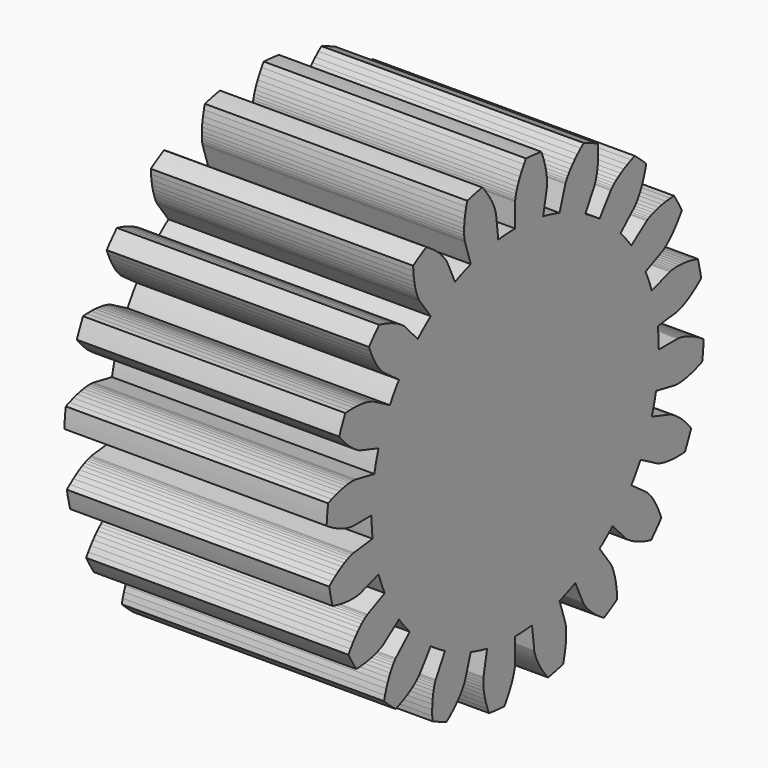
from build123d import *

# Parameters (mm, degrees)
F2_DEPTH = 12.7


# Not quite as in the source:
# - a variable given as a bare number and used for a length is read in inches; the dataset says mm whatever the document's units were


with BuildPart() as f2:
    # F1 (on Right) → F2 (new body)
    with BuildSketch(Plane.YZ):
        with BuildLine():
            ThreePointArc((8.5236223657, -1.6954539034), (8.6487623375, -0.8518287399), (8.69061, 0))
            ThreePointArc((8.69061, 0), (8.6755370945, 0.5116231949), (8.6303706627, 1.0214716817))
            ThreePointArc((8.6303706627, 1.0214716817), (8.4886913359, 1.8624772687), (8.2652612711, 2.6855461815))
            ThreePointArc((8.2652612711, 2.6855461815), (8.0928258242, 3.167470971), (7.8923181479, 3.6384085016))
            ThreePointArc((7.8923181479, 3.6384085016), (7.4976880821, 4.3944710257), (7.0308511815, 5.1082123914))
            ThreePointArc((7.0308511815, 5.1082123914), (6.7179323761, 5.5132646193), (6.3817105437, 5.8991925471))
            ThreePointArc((6.3817105437, 5.8991925471), (5.7727588794, 6.4963033405), (5.1082123914, 7.0308511815))
            ThreePointArc((5.1082123914, 7.0308511815), (4.6854409005, 7.3193815135), (4.2464166476, 7.582522524))
            ThreePointArc((4.2464166476, 7.582522524), (3.4827518165, 7.962232222), (2.6855461815, 8.2652612711))
            ThreePointArc((2.6855461815, 8.2652612711), (2.1943058241, 8.4090263481), (1.6954539034, 8.5236223657))
            ThreePointArc((1.6954539034, 8.5236223657), (0.8518287399, 8.6487623375), (0, 8.69061))
            ThreePointArc((0, 8.69061), (-0.5116231949, 8.6755370945), (-1.0214716817, 8.6303706627))
            ThreePointArc((-1.0214716817, 8.6303706627), (-1.8624772687, 8.4886913359), (-2.6855461815, 8.2652612711))
            ThreePointArc((-2.6855461815, 8.2652612711), (-3.167470971, 8.0928258242), (-3.6384085016, 7.8923181479))
            ThreePointArc((-3.6384085016, 7.8923181479), (-4.3944710257, 7.4976880821), (-5.1082123914, 7.0308511815))
            ThreePointArc((-5.1082123914, 7.0308511815), (-5.5132646193, 6.7179323761), (-5.8991925471, 6.3817105437))
            ThreePointArc((-5.8991925471, 6.3817105437), (-6.4963033405, 5.7727588794), (-7.0308511815, 5.1082123914))
            ThreePointArc((-7.0308511815, 5.1082123914), (-7.3193815135, 4.6854409005), (-7.582522524, 4.2464166476))
            ThreePointArc((-7.582522524, 4.2464166476), (-7.962232222, 3.4827518165), (-8.2652612711, 2.6855461815))
            ThreePointArc((-8.2652612711, 2.6855461815), (-8.4090263481, 2.1943058241), (-8.5236223657, 1.6954539034))
            ThreePointArc((-8.5236223657, 1.6954539034), (-8.6487623375, 0.8518287399), (-8.69061, 0))
            ThreePointArc((-8.69061, 0), (-8.6755370945, -0.5116231949), (-8.6303706627, -1.0214716817))
            ThreePointArc((-8.6303706627, -1.0214716817), (-8.4886913359, -1.8624772687), (-8.2652612711, -2.6855461815))
            ThreePointArc((-8.2652612711, -2.6855461815), (-8.0928258242, -3.167470971), (-7.8923181479, -3.6384085016))
            ThreePointArc((-7.8923181479, -3.6384085016), (-7.4976880821, -4.3944710257), (-7.0308511815, -5.1082123914))
            ThreePointArc((-7.0308511815, -5.1082123914), (-6.7179323761, -5.5132646193), (-6.3817105437, -5.8991925471))
            ThreePointArc((-6.3817105437, -5.8991925471), (-5.7727588794, -6.4963033405), (-5.1082123914, -7.0308511815))
            ThreePointArc((-5.1082123914, -7.0308511815), (-4.6854409005, -7.3193815135), (-4.2464166476, -7.582522524))
            ThreePointArc((-4.2464166476, -7.582522524), (-3.4827518165, -7.962232222), (-2.6855461815, -8.2652612711))
            ThreePointArc((-2.6855461815, -8.2652612711), (-2.1943058241, -8.4090263481), (-1.6954539034, -8.5236223657))
            ThreePointArc((-1.6954539034, -8.5236223657), (-0.8518287399, -8.6487623375), (0, -8.69061))
            ThreePointArc((0, -8.69061), (0.5116231949, -8.6755370945), (1.0214716817, -8.6303706627))
            ThreePointArc((1.0214716817, -8.6303706627), (1.8624772687, -8.4886913359), (2.6855461815, -8.2652612711))
            ThreePointArc((2.6855461815, -8.2652612711), (3.167470971, -8.0928258242), (3.6384085016, -7.8923181479))
            ThreePointArc((3.6384085016, -7.8923181479), (4.3944710257, -7.4976880821), (5.1082123914, -7.0308511815))
            ThreePointArc((5.1082123914, -7.0308511815), (5.5132646193, -6.7179323761), (5.8991925471, -6.3817105437))
            ThreePointArc((5.8991925471, -6.3817105437), (6.4963033405, -5.7727588794), (7.0308511815, -5.1082123914))
            ThreePointArc((7.0308511815, -5.1082123914), (7.3193815135, -4.6854409005), (7.582522524, -4.2464166476))
            ThreePointArc((7.582522524, -4.2464166476), (7.962232222, -3.4827518165), (8.2652612711, -2.6855461815))
            ThreePointArc((8.2652612711, -2.6855461815), (8.4090263481, -2.1943058241), (8.5236223657, -1.6954539034))
        make_face()
        with BuildLine():
            Line((-9.3549533207, -3.0396085912), (-8.2652612711, -2.6855461815))
            ThreePointArc((-8.2652612711, -2.6855461815), (-8.4886913359, -1.8624772687), (-8.6303706627, -1.0214716817))
            Line((-8.6303706627, -1.0214716817), (-9.7681987347, -1.1561425087))
            Line((-9.7681987347, -1.1561425087), (-9.780353193, -1.157993683))
            Line((-9.780353193, -1.157993683), (-9.8165326998, -1.1651615743))
            Line((-9.8165326998, -1.1651615743), (-9.8761758653, -1.180040537))
            Line((-9.8761758653, -1.180040537), (-9.9585426782, -1.2049790988))
            Line((-9.9585426782, -1.2049790988), (-10.0627178322, -1.2422681281))
            Line((-10.0627178322, -1.2422681281), (-10.1876147871, -1.2941292255))
            Line((-10.1876147871, -1.2941292255), (-10.3319805495, -1.3627033855))
            Line((-10.3319805495, -1.3627033855), (-10.4944011563, -1.4500399701))
            Line((-10.4944011563, -1.4500399701), (-10.6733078407, -1.5580860349))
            Line((-10.6733078407, -1.5580860349), (-10.8669838603, -1.6886760511))
            Line((-10.8669838603, -1.6886760511), (-11.0735719609, -1.8435220595))
            Line((-11.0735719609, -1.8435220595), (-11.2547256997, -1.994003366))
            ThreePointArc((-11.2547256997, -1.994003366), (-11.1644340235, -2.4495536195), (-11.0557112434, -2.901059962))
            Line((-11.0557112434, -2.901059962), (-10.8281972477, -2.9618767566))
            Line((-10.8281972477, -2.9618767566), (-10.5757578852, -3.0160089821))
            Line((-10.5757578852, -3.0160089821), (-10.3451995481, -3.0535190624))
            Line((-10.3451995481, -3.0535190624), (-10.1374921268, -3.0767393331))
            Line((-10.1374921268, -3.0767393331), (-9.9534266499, -3.0880544876))
            Line((-9.9534266499, -3.0880544876), (-9.7936126283, -3.0898895107))
            Line((-9.7936126283, -3.0898895107), (-9.6584761579, -3.0846974859))
            Line((-9.6584761579, -3.0846974859), (-9.5482587877, -3.0749473207))
            Line((-9.5482587877, -3.0749473207), (-9.4630171571, -3.0631114372))
            Line((-9.4630171571, -3.0631114372), (-9.4026234009, -3.0516534735))
            Line((-9.4026234009, -3.0516534735), (-9.3667663213, -3.0430160422))
            Line((-9.3667663213, -3.0430160422), (-9.3549533207, -3.0396085912))
        make_face()
        with BuildLine():
            Line((-7.9577986044, -5.7816791154), (-7.0308511815, -5.1082123914))
            ThreePointArc((-7.0308511815, -5.1082123914), (-7.4976880821, -4.3944710257), (-7.8923181479, -3.6384085016))
            Line((-7.8923181479, -3.6384085016), (-8.932841376, -4.1180962801))
            Line((-8.932841376, -4.1180962801), (-8.9438289085, -4.1236127857))
            Line((-8.9438289085, -4.1236127857), (-8.9760226639, -4.1416099379))
            Line((-8.9760226639, -4.1416099379), (-9.0281488328, -4.174191424))
            Line((-9.0281488328, -4.174191424), (-9.0987778875, -4.2233621507))
            Line((-9.0987778875, -4.2233621507), (-9.1863314028, -4.291018018))
            Line((-9.1863314028, -4.291018018), (-9.2890895052, -4.3789361342))
            Line((-9.2890895052, -4.3789361342), (-9.4051989235, -4.4887655099))
            Line((-9.4051989235, -4.4887655099), (-9.532681611, -4.6220182655))
            Line((-9.532681611, -4.6220182655), (-9.6694439088, -4.7800613854))
            Line((-9.6694439088, -4.7800613854), (-9.813286215, -4.9641090528))
            Line((-9.813286215, -4.9641090528), (-9.9619131262, -5.175215592))
            Line((-9.9619131262, -5.175215592), (-10.0876992889, -5.374311403))
            ThreePointArc((-10.0876992889, -5.374311403), (-9.8610540317, -5.7796637777), (-9.6181293903, -6.1754746402))
            Line((-9.6181293903, -6.1754746402), (-9.3829572991, -6.1630091578))
            Line((-9.3829572991, -6.1630091578), (-9.1261454208, -6.1364839106))
            Line((-9.1261454208, -6.1364839106), (-8.8952801597, -6.1009116725))
            Line((-8.8952801597, -6.1009116725), (-8.6905632048, -6.0588103392))
            Line((-8.6905632048, -6.0588103392), (-8.5120099586, -6.0126923302))
            Line((-8.5120099586, -6.0126923302), (-8.3594507387, -5.9650522923))
            Line((-8.3594507387, -5.9650522923), (-8.2325327418, -5.9183549173))
            Line((-8.2325327418, -5.9183549173), (-8.1307227604, -5.8750229187))
            Line((-8.1307227604, -5.8750229187), (-8.0533106413, -5.837425212))
            Line((-8.0533106413, -5.837425212), (-7.9994134714, -5.807865344))
            Line((-7.9994134714, -5.807865344), (-7.9679804752, -5.7885702118))
            Line((-7.9679804752, -5.7885702118), (-7.9577986044, -5.7816791154))
        make_face()
        with BuildLine():
            Line((-5.7816791154, -7.9577986044), (-5.1082123914, -7.0308511815))
            ThreePointArc((-5.1082123914, -7.0308511815), (-5.7727588794, -6.4963033405), (-6.3817105437, -5.8991925471))
            Line((-6.3817105437, -5.8991925471), (-7.2230752646, -6.6769420952))
            Line((-7.2230752646, -6.6769420952), (-7.231820335, -6.685583938))
            Line((-7.231820335, -6.685583938), (-7.2568769901, -6.7126486644))
            Line((-7.2568769901, -6.7126486644), (-7.2963836897, -6.7597433711))
            Line((-7.2963836897, -6.7597433711), (-7.3483613222, -6.8283330894))
            Line((-7.3483613222, -6.8283330894), (-7.4107228507, -6.9197331669))
            Line((-7.4107228507, -6.9197331669), (-7.4812834216, -7.0351022642))
            Line((-7.4812834216, -7.0351022642), (-7.5577708969, -7.1754359912))
            Line((-7.5577708969, -7.1754359912), (-7.6378367716, -7.3415612096))
            Line((-7.6378367716, -7.3415612096), (-7.7190674362, -7.5341310229))
            Line((-7.7190674362, -7.5341310229), (-7.7989957418, -7.7536204733))
            Line((-7.7989957418, -7.7536204733), (-7.8751128259, -8.0003229645))
            Line((-7.8751128259, -8.0003229645), (-7.9332185865, -8.2285443949))
            ThreePointArc((-7.9332185865, -8.2285443949), (-7.5924053653, -8.544020176), (-7.2390580191, -8.8453908334))
            Line((-7.2390580191, -8.8453908334), (-7.0192481152, -8.7608632825))
            Line((-7.0192481152, -8.7608632825), (-6.783202257, -8.6562770384))
            Line((-6.783202257, -8.6562770384), (-6.5746287721, -8.5511045405))
            Line((-6.5746287721, -8.5511045405), (-6.3929414057, -8.4478027751))
            Line((-6.3929414057, -8.4478027751), (-6.2373784259, -8.3487659546))
            Line((-6.2373784259, -8.3487659546), (-6.107007567, -8.2563141945))
            Line((-6.107007567, -8.2563141945), (-6.0007316615, -8.1726825338))
            Line((-6.0007316615, -8.1726825338), (-5.9172949393, -8.1000103397))
            Line((-5.9172949393, -8.1000103397), (-5.8552899692, -8.0403311354))
            Line((-5.8552899692, -8.0403311354), (-5.8131652162, -7.9955628889))
            Line((-5.8131652162, -7.9955628889), (-5.7892331841, -7.9674987976))
            Line((-5.7892331841, -7.9674987976), (-5.7816791154, -7.9577986044))
        make_face()
        with BuildLine():
            Line((-3.0396085912, -9.3549533207), (-2.6855461815, -8.2652612711))
            ThreePointArc((-2.6855461815, -8.2652612711), (-3.4827518165, -7.962232222), (-4.2464166476, -7.582522524))
            Line((-4.2464166476, -7.582522524), (-4.8062642203, -8.5822022969))
            Line((-4.8062642203, -8.5822022969), (-4.8119108001, -8.5931235533))
            Line((-4.8119108001, -8.5931235533), (-4.8273776348, -8.6266065699))
            Line((-4.8273776348, -8.6266065699), (-4.8503976742, -8.6836045392))
            Line((-4.8503976742, -8.6836045392), (-4.8786359517, -8.7648992095))
            Line((-4.8786359517, -8.7648992095), (-4.9097011125, -8.8710966209))
            Line((-4.9097011125, -8.8710966209), (-4.9411571916, -9.0026235682))
            Line((-4.9411571916, -9.0026235682), (-4.9705355968, -9.1597248034))
            Line((-4.9705355968, -9.1597248034), (-4.995347253, -9.3424609909))
            Line((-4.995347253, -9.3424609909), (-5.013094861, -9.5507074225))
            Line((-5.013094861, -9.5507074225), (-5.0212852266, -9.7841534993))
            Line((-5.0212852266, -9.7841534993), (-5.0174416132, -10.0423029836))
            Line((-5.0174416132, -10.0423029836), (-5.0021791749, -10.2773101297))
            ThreePointArc((-5.0021791749, -10.2773101297), (-4.5805591624, -10.4720283498), (-4.1513772115, -10.6494585425))
            Line((-4.1513772115, -10.6494585425), (-3.9684460198, -10.5011430685))
            Line((-3.9684460198, -10.5011430685), (-3.776271995, -10.328733458))
            Line((-3.776271995, -10.328733458), (-3.6104069123, -10.1642557171))
            Line((-3.6104069123, -10.1642557171), (-3.4695339596, -10.009865416))
            Line((-3.4695339596, -10.009865416), (-3.3521888346, -9.8676041981))
            Line((-3.3521888346, -9.8676041981), (-3.2567679447, -9.7393905383))
            Line((-3.2567679447, -9.7393905383), (-3.1815371566, -9.6270110415))
            Line((-3.1815371566, -9.6270110415), (-3.1246410612, -9.5321123126))
            Line((-3.1246410612, -9.5321123126), (-3.0841127188, -9.456193427))
            Line((-3.0841127188, -9.456193427), (-3.0578838469, -9.4005990298))
            Line((-3.0578838469, -9.4005990298), (-3.043795413, -9.3665130884))
            Line((-3.043795413, -9.3665130884), (-3.0396085912, -9.3549533207))
        make_face()
        with BuildLine():
            Line((0, -9.8363800262), (0, -8.69061))
            ThreePointArc((0, -8.69061), (-0.8518287399, -8.6487623375), (-1.6954539034, -8.5236223657))
            Line((-1.6954539034, -8.5236223657), (-1.9189825468, -9.6473767422))
            Line((-1.9189825468, -9.6473767422), (-1.9209779096, -9.6595083634))
            Line((-1.9209779096, -9.6595083634), (-1.9253409223, -9.6961321192))
            Line((-1.9253409223, -9.6961321192), (-1.9296209396, -9.7574539927))
            Line((-1.9296209396, -9.7574539927), (-1.9313557028, -9.8434959263))
            Line((-1.9313557028, -9.8434959263), (-1.9280836215, -9.9540953291))
            Line((-1.9280836215, -9.9540953291), (-1.9173560686, -10.0889053524))
            Line((-1.9173560686, -10.0889053524), (-1.8967496408, -10.2473959323))
            Line((-1.8967496408, -10.2473959323), (-1.8638783407, -10.4288555976))
            Line((-1.8638783407, -10.4288555976), (-1.8164056325, -10.6323940358))
            Line((-1.8164056325, -10.6323940358), (-1.7520563281, -10.8569454106))
            Line((-1.7520563281, -10.8569454106), (-1.6686282567, -11.101272418))
            Line((-1.6686282567, -11.101272418), (-1.5814916135, -11.3200611428))
            ThreePointArc((-1.5814916135, -11.3200611428), (-1.120335914, -11.3749614259), (-0.657330678, -11.4110830503))
            Line((-0.657330678, -11.4110830503), (-0.5291847781, -11.2134978052))
            Line((-0.5291847781, -11.2134978052), (-0.3996939192, -10.9901414821))
            Line((-0.3996939192, -10.9901414821), (-0.2927732686, -10.7824587255))
            Line((-0.2927732686, -10.7824587255), (-0.2065043558, -10.5920926872))
            Line((-0.2065043558, -10.5920926872), (-0.138863644, -10.4205325911))
            Line((-0.138863644, -10.4205325911), (-0.0877331847, -10.2691074778))
            Line((-0.0877331847, -10.2691074778), (-0.0509116278, -10.1389806331))
            Line((-0.0509116278, -10.1389806331), (-0.0261255455, -10.0311447182))
            Line((-0.0261255455, -10.0311447182), (-0.0110410272, -9.9464176208))
            Line((-0.0110410272, -9.9464176208), (-0.0032755011, -9.8854390399))
            Line((-0.0032755011, -9.8854390399), (-0.0004097394, -9.8486678177))
            Line((-0.0004097394, -9.8486678177), (0, -9.8363800262))
        make_face()
        with BuildLine():
            Line((3.0396085912, -9.3549533207), (2.6855461815, -8.2652612711))
            ThreePointArc((2.6855461815, -8.2652612711), (1.8624772687, -8.4886913359), (1.0214716817, -8.6303706627))
            Line((1.0214716817, -8.6303706627), (1.1561425087, -9.7681987347))
            Line((1.1561425087, -9.7681987347), (1.157993683, -9.780353193))
            Line((1.157993683, -9.780353193), (1.1651615743, -9.8165326998))
            Line((1.1651615743, -9.8165326998), (1.180040537, -9.8761758653))
            Line((1.180040537, -9.8761758653), (1.2049790988, -9.9585426782))
            Line((1.2049790988, -9.9585426782), (1.2422681281, -10.0627178322))
            Line((1.2422681281, -10.0627178322), (1.2941292255, -10.1876147871))
            Line((1.2941292255, -10.1876147871), (1.3627033855, -10.3319805495))
            Line((1.3627033855, -10.3319805495), (1.4500399701, -10.4944011563))
            Line((1.4500399701, -10.4944011563), (1.5580860349, -10.6733078407))
            Line((1.5580860349, -10.6733078407), (1.6886760511, -10.8669838603))
            Line((1.6886760511, -10.8669838603), (1.8435220595, -11.0735719609))
            Line((1.8435220595, -11.0735719609), (1.994003366, -11.2547256997))
            ThreePointArc((1.994003366, -11.2547256997), (2.4495536195, -11.1644340235), (2.901059962, -11.0557112434))
            Line((2.901059962, -11.0557112434), (2.9618767566, -10.8281972477))
            Line((2.9618767566, -10.8281972477), (3.0160089821, -10.5757578852))
            Line((3.0160089821, -10.5757578852), (3.0535190624, -10.3451995481))
            Line((3.0535190624, -10.3451995481), (3.0767393331, -10.1374921268))
            Line((3.0767393331, -10.1374921268), (3.0880544876, -9.9534266499))
            Line((3.0880544876, -9.9534266499), (3.0898895107, -9.7936126283))
            Line((3.0898895107, -9.7936126283), (3.0846974859, -9.6584761579))
            Line((3.0846974859, -9.6584761579), (3.0749473207, -9.5482587877))
            Line((3.0749473207, -9.5482587877), (3.0631114372, -9.4630171571))
            Line((3.0631114372, -9.4630171571), (3.0516534735, -9.4026234009))
            Line((3.0516534735, -9.4026234009), (3.0430160422, -9.3667663213))
            Line((3.0430160422, -9.3667663213), (3.0396085912, -9.3549533207))
        make_face()
        with BuildLine():
            Line((5.7816791154, -7.9577986044), (5.1082123914, -7.0308511815))
            ThreePointArc((5.1082123914, -7.0308511815), (4.3944710257, -7.4976880821), (3.6384085016, -7.8923181479))
            Line((3.6384085016, -7.8923181479), (4.1180962801, -8.932841376))
            Line((4.1180962801, -8.932841376), (4.1236127857, -8.9438289085))
            Line((4.1236127857, -8.9438289085), (4.1416099379, -8.9760226639))
            Line((4.1416099379, -8.9760226639), (4.174191424, -9.0281488328))
            Line((4.174191424, -9.0281488328), (4.2233621507, -9.0987778875))
            Line((4.2233621507, -9.0987778875), (4.291018018, -9.1863314028))
            Line((4.291018018, -9.1863314028), (4.3789361342, -9.2890895052))
            Line((4.3789361342, -9.2890895052), (4.4887655099, -9.4051989235))
            Line((4.4887655099, -9.4051989235), (4.6220182655, -9.532681611))
            Line((4.6220182655, -9.532681611), (4.7800613854, -9.6694439088))
            Line((4.7800613854, -9.6694439088), (4.9641090528, -9.813286215))
            Line((4.9641090528, -9.813286215), (5.175215592, -9.9619131262))
            Line((5.175215592, -9.9619131262), (5.374311403, -10.0876992889))
            ThreePointArc((5.374311403, -10.0876992889), (5.7796637777, -9.8610540317), (6.1754746402, -9.6181293903))
            Line((6.1754746402, -9.6181293903), (6.1630091578, -9.3829572991))
            Line((6.1630091578, -9.3829572991), (6.1364839106, -9.1261454208))
            Line((6.1364839106, -9.1261454208), (6.1009116725, -8.8952801597))
            Line((6.1009116725, -8.8952801597), (6.0588103392, -8.6905632048))
            Line((6.0588103392, -8.6905632048), (6.0126923302, -8.5120099586))
            Line((6.0126923302, -8.5120099586), (5.9650522923, -8.3594507387))
            Line((5.9650522923, -8.3594507387), (5.9183549173, -8.2325327418))
            Line((5.9183549173, -8.2325327418), (5.8750229187, -8.1307227604))
            Line((5.8750229187, -8.1307227604), (5.837425212, -8.0533106413))
            Line((5.837425212, -8.0533106413), (5.807865344, -7.9994134714))
            Line((5.807865344, -7.9994134714), (5.7885702118, -7.9679804752))
            Line((5.7885702118, -7.9679804752), (5.7816791154, -7.9577986044))
        make_face()
        with BuildLine():
            Line((7.9577986044, -5.7816791154), (7.0308511815, -5.1082123914))
            ThreePointArc((7.0308511815, -5.1082123914), (6.4963033405, -5.7727588794), (5.8991925471, -6.3817105437))
            Line((5.8991925471, -6.3817105437), (6.6769420952, -7.2230752646))
            Line((6.6769420952, -7.2230752646), (6.685583938, -7.231820335))
            Line((6.685583938, -7.231820335), (6.7126486644, -7.2568769901))
            Line((6.7126486644, -7.2568769901), (6.7597433711, -7.2963836897))
            Line((6.7597433711, -7.2963836897), (6.8283330894, -7.3483613222))
            Line((6.8283330894, -7.3483613222), (6.9197331669, -7.4107228507))
            Line((6.9197331669, -7.4107228507), (7.0351022642, -7.4812834216))
            Line((7.0351022642, -7.4812834216), (7.1754359912, -7.5577708969))
            Line((7.1754359912, -7.5577708969), (7.3415612096, -7.6378367716))
            Line((7.3415612096, -7.6378367716), (7.5341310229, -7.7190674362))
            Line((7.5341310229, -7.7190674362), (7.7536204733, -7.7989957418))
            Line((7.7536204733, -7.7989957418), (8.0003229645, -7.8751128259))
            Line((8.0003229645, -7.8751128259), (8.2285443949, -7.9332185865))
            ThreePointArc((8.2285443949, -7.9332185865), (8.544020176, -7.5924053653), (8.8453908334, -7.2390580191))
            Line((8.8453908334, -7.2390580191), (8.7608632825, -7.0192481152))
            Line((8.7608632825, -7.0192481152), (8.6562770384, -6.783202257))
            Line((8.6562770384, -6.783202257), (8.5511045405, -6.5746287721))
            Line((8.5511045405, -6.5746287721), (8.4478027751, -6.3929414057))
            Line((8.4478027751, -6.3929414057), (8.3487659546, -6.2373784259))
            Line((8.3487659546, -6.2373784259), (8.2563141945, -6.107007567))
            Line((8.2563141945, -6.107007567), (8.1726825338, -6.0007316615))
            Line((8.1726825338, -6.0007316615), (8.1000103397, -5.9172949393))
            Line((8.1000103397, -5.9172949393), (8.0403311354, -5.8552899692))
            Line((8.0403311354, -5.8552899692), (7.9955628889, -5.8131652162))
            Line((7.9955628889, -5.8131652162), (7.9674987976, -5.7892331841))
            Line((7.9674987976, -5.7892331841), (7.9577986044, -5.7816791154))
        make_face()
        with BuildLine():
            Line((9.3549533207, -3.0396085912), (8.2652612711, -2.6855461815))
            ThreePointArc((8.2652612711, -2.6855461815), (7.962232222, -3.4827518165), (7.582522524, -4.2464166476))
            Line((7.582522524, -4.2464166476), (8.5822022969, -4.8062642203))
            Line((8.5822022969, -4.8062642203), (8.5931235533, -4.8119108001))
            Line((8.5931235533, -4.8119108001), (8.6266065699, -4.8273776348))
            Line((8.6266065699, -4.8273776348), (8.6836045392, -4.8503976742))
            Line((8.6836045392, -4.8503976742), (8.7648992095, -4.8786359517))
            Line((8.7648992095, -4.8786359517), (8.8710966209, -4.9097011125))
            Line((8.8710966209, -4.9097011125), (9.0026235682, -4.9411571916))
            Line((9.0026235682, -4.9411571916), (9.1597248034, -4.9705355968))
            Line((9.1597248034, -4.9705355968), (9.3424609909, -4.995347253))
            Line((9.3424609909, -4.995347253), (9.5507074225, -5.013094861))
            Line((9.5507074225, -5.013094861), (9.7841534993, -5.0212852266))
            Line((9.7841534993, -5.0212852266), (10.0423029836, -5.0174416132))
            Line((10.0423029836, -5.0174416132), (10.2773101297, -5.0021791749))
            ThreePointArc((10.2773101297, -5.0021791749), (10.4720283498, -4.5805591624), (10.6494585425, -4.1513772115))
            Line((10.6494585425, -4.1513772115), (10.5011430685, -3.9684460198))
            Line((10.5011430685, -3.9684460198), (10.328733458, -3.776271995))
            Line((10.328733458, -3.776271995), (10.1642557171, -3.6104069123))
            Line((10.1642557171, -3.6104069123), (10.009865416, -3.4695339596))
            Line((10.009865416, -3.4695339596), (9.8676041981, -3.3521888346))
            Line((9.8676041981, -3.3521888346), (9.7393905383, -3.2567679447))
            Line((9.7393905383, -3.2567679447), (9.6270110415, -3.1815371566))
            Line((9.6270110415, -3.1815371566), (9.5321123126, -3.1246410612))
            Line((9.5321123126, -3.1246410612), (9.456193427, -3.0841127188))
            Line((9.456193427, -3.0841127188), (9.4005990298, -3.0578838469))
            Line((9.4005990298, -3.0578838469), (9.3665130884, -3.043795413))
            Line((9.3665130884, -3.043795413), (9.3549533207, -3.0396085912))
        make_face()
        with BuildLine():
            Line((9.8363800262, 0), (8.69061, 0))
            ThreePointArc((8.69061, 0), (8.6487623375, -0.8518287399), (8.5236223657, -1.6954539034))
            Line((8.5236223657, -1.6954539034), (9.6473767422, -1.9189825468))
            Line((9.6473767422, -1.9189825468), (9.6595083634, -1.9209779096))
            Line((9.6595083634, -1.9209779096), (9.6961321192, -1.9253409223))
            Line((9.6961321192, -1.9253409223), (9.7574539927, -1.9296209396))
            Line((9.7574539927, -1.9296209396), (9.8434959263, -1.9313557028))
            Line((9.8434959263, -1.9313557028), (9.9540953291, -1.9280836215))
            Line((9.9540953291, -1.9280836215), (10.0889053524, -1.9173560686))
            Line((10.0889053524, -1.9173560686), (10.2473959323, -1.8967496408))
            Line((10.2473959323, -1.8967496408), (10.4288555976, -1.8638783407))
            Line((10.4288555976, -1.8638783407), (10.6323940358, -1.8164056325))
            Line((10.6323940358, -1.8164056325), (10.8569454106, -1.7520563281))
            Line((10.8569454106, -1.7520563281), (11.101272418, -1.6686282567))
            Line((11.101272418, -1.6686282567), (11.3200611428, -1.5814916135))
            ThreePointArc((11.3200611428, -1.5814916135), (11.3749614259, -1.120335914), (11.4110830503, -0.657330678))
            Line((11.4110830503, -0.657330678), (11.2134978052, -0.5291847781))
            Line((11.2134978052, -0.5291847781), (10.9901414821, -0.3996939192))
            Line((10.9901414821, -0.3996939192), (10.7824587255, -0.2927732686))
            Line((10.7824587255, -0.2927732686), (10.5920926872, -0.2065043558))
            Line((10.5920926872, -0.2065043558), (10.4205325911, -0.138863644))
            Line((10.4205325911, -0.138863644), (10.2691074778, -0.0877331847))
            Line((10.2691074778, -0.0877331847), (10.1389806331, -0.0509116278))
            Line((10.1389806331, -0.0509116278), (10.0311447182, -0.0261255455))
            Line((10.0311447182, -0.0261255455), (9.9464176208, -0.0110410272))
            Line((9.9464176208, -0.0110410272), (9.8854390399, -0.0032755011))
            Line((9.8854390399, -0.0032755011), (9.8486678177, -0.0004097394))
            Line((9.8486678177, -0.0004097394), (9.8363800262, 0))
        make_face()
        with BuildLine():
            ThreePointArc((8.2652612711, 2.6855461815), (8.4886913359, 1.8624772687), (8.6303706627, 1.0214716817))
            Line((8.6303706627, 1.0214716817), (9.7681987347, 1.1561425087))
            Line((9.7681987347, 1.1561425087), (9.780353193, 1.157993683))
            Line((9.780353193, 1.157993683), (9.8165326998, 1.1651615743))
            Line((9.8165326998, 1.1651615743), (9.8761758653, 1.180040537))
            Line((9.8761758653, 1.180040537), (9.9585426782, 1.2049790988))
            Line((9.9585426782, 1.2049790988), (10.0627178322, 1.2422681281))
            Line((10.0627178322, 1.2422681281), (10.1876147871, 1.2941292255))
            Line((10.1876147871, 1.2941292255), (10.3319805495, 1.3627033855))
            Line((10.3319805495, 1.3627033855), (10.4944011563, 1.4500399701))
            Line((10.4944011563, 1.4500399701), (10.6733078407, 1.5580860349))
            Line((10.6733078407, 1.5580860349), (10.8669838603, 1.6886760511))
            Line((10.8669838603, 1.6886760511), (11.0735719609, 1.8435220595))
            Line((11.0735719609, 1.8435220595), (11.2547256997, 1.994003366))
            ThreePointArc((11.2547256997, 1.994003366), (11.1644340235, 2.4495536195), (11.0557112434, 2.901059962))
            Line((11.0557112434, 2.901059962), (10.8281972477, 2.9618767566))
            Line((10.8281972477, 2.9618767566), (10.5757578852, 3.0160089821))
            Line((10.5757578852, 3.0160089821), (10.3451995481, 3.0535190624))
            Line((10.3451995481, 3.0535190624), (10.1374921268, 3.0767393331))
            Line((10.1374921268, 3.0767393331), (9.9534266499, 3.0880544876))
            Line((9.9534266499, 3.0880544876), (9.7936126283, 3.0898895107))
            Line((9.7936126283, 3.0898895107), (9.6584761579, 3.0846974859))
            Line((9.6584761579, 3.0846974859), (9.5482587877, 3.0749473207))
            Line((9.5482587877, 3.0749473207), (9.4630171571, 3.0631114372))
            Line((9.4630171571, 3.0631114372), (9.4026234009, 3.0516534735))
            Line((9.4026234009, 3.0516534735), (9.3667663213, 3.0430160422))
            Line((9.3667663213, 3.0430160422), (9.3549533207, 3.0396085912))
            Line((9.3549533207, 3.0396085912), (8.2652612711, 2.6855461815))
        make_face()
        with BuildLine():
            ThreePointArc((7.0308511815, 5.1082123914), (7.4976880821, 4.3944710257), (7.8923181479, 3.6384085016))
            Line((7.8923181479, 3.6384085016), (8.932841376, 4.1180962801))
            Line((8.932841376, 4.1180962801), (8.9438289085, 4.1236127857))
            Line((8.9438289085, 4.1236127857), (8.9760226639, 4.1416099379))
            Line((8.9760226639, 4.1416099379), (9.0281488328, 4.174191424))
            Line((9.0281488328, 4.174191424), (9.0987778875, 4.2233621507))
            Line((9.0987778875, 4.2233621507), (9.1863314028, 4.291018018))
            Line((9.1863314028, 4.291018018), (9.2890895052, 4.3789361342))
            Line((9.2890895052, 4.3789361342), (9.4051989235, 4.4887655099))
            Line((9.4051989235, 4.4887655099), (9.532681611, 4.6220182655))
            Line((9.532681611, 4.6220182655), (9.6694439088, 4.7800613854))
            Line((9.6694439088, 4.7800613854), (9.813286215, 4.9641090528))
            Line((9.813286215, 4.9641090528), (9.9619131262, 5.175215592))
            Line((9.9619131262, 5.175215592), (10.0876992889, 5.374311403))
            ThreePointArc((10.0876992889, 5.374311403), (9.8610540317, 5.7796637777), (9.6181293903, 6.1754746402))
            Line((9.6181293903, 6.1754746402), (9.3829572991, 6.1630091578))
            Line((9.3829572991, 6.1630091578), (9.1261454208, 6.1364839106))
            Line((9.1261454208, 6.1364839106), (8.8952801597, 6.1009116725))
            Line((8.8952801597, 6.1009116725), (8.6905632048, 6.0588103392))
            Line((8.6905632048, 6.0588103392), (8.5120099586, 6.0126923302))
            Line((8.5120099586, 6.0126923302), (8.3594507387, 5.9650522923))
            Line((8.3594507387, 5.9650522923), (8.2325327418, 5.9183549173))
            Line((8.2325327418, 5.9183549173), (8.1307227604, 5.8750229187))
            Line((8.1307227604, 5.8750229187), (8.0533106413, 5.837425212))
            Line((8.0533106413, 5.837425212), (7.9994134714, 5.807865344))
            Line((7.9994134714, 5.807865344), (7.9679804752, 5.7885702118))
            Line((7.9679804752, 5.7885702118), (7.9577986044, 5.7816791154))
            Line((7.9577986044, 5.7816791154), (7.0308511815, 5.1082123914))
        make_face()
        with BuildLine():
            ThreePointArc((5.1082123914, 7.0308511815), (5.7727588794, 6.4963033405), (6.3817105437, 5.8991925471))
            Line((6.3817105437, 5.8991925471), (7.2230752646, 6.6769420952))
            Line((7.2230752646, 6.6769420952), (7.231820335, 6.685583938))
            Line((7.231820335, 6.685583938), (7.2568769901, 6.7126486644))
            Line((7.2568769901, 6.7126486644), (7.2963836897, 6.7597433711))
            Line((7.2963836897, 6.7597433711), (7.3483613222, 6.8283330894))
            Line((7.3483613222, 6.8283330894), (7.4107228507, 6.9197331669))
            Line((7.4107228507, 6.9197331669), (7.4812834216, 7.0351022642))
            Line((7.4812834216, 7.0351022642), (7.5577708969, 7.1754359912))
            Line((7.5577708969, 7.1754359912), (7.6378367716, 7.3415612096))
            Line((7.6378367716, 7.3415612096), (7.7190674362, 7.5341310229))
            Line((7.7190674362, 7.5341310229), (7.7989957418, 7.7536204733))
            Line((7.7989957418, 7.7536204733), (7.8751128259, 8.0003229645))
            Line((7.8751128259, 8.0003229645), (7.9332185865, 8.2285443949))
            ThreePointArc((7.9332185865, 8.2285443949), (7.5924053653, 8.544020176), (7.2390580191, 8.8453908334))
            Line((7.2390580191, 8.8453908334), (7.0192481152, 8.7608632825))
            Line((7.0192481152, 8.7608632825), (6.783202257, 8.6562770384))
            Line((6.783202257, 8.6562770384), (6.5746287721, 8.5511045405))
            Line((6.5746287721, 8.5511045405), (6.3929414057, 8.4478027751))
            Line((6.3929414057, 8.4478027751), (6.2373784259, 8.3487659546))
            Line((6.2373784259, 8.3487659546), (6.107007567, 8.2563141945))
            Line((6.107007567, 8.2563141945), (6.0007316615, 8.1726825338))
            Line((6.0007316615, 8.1726825338), (5.9172949393, 8.1000103397))
            Line((5.9172949393, 8.1000103397), (5.8552899692, 8.0403311354))
            Line((5.8552899692, 8.0403311354), (5.8131652162, 7.9955628889))
            Line((5.8131652162, 7.9955628889), (5.7892331841, 7.9674987976))
            Line((5.7892331841, 7.9674987976), (5.7816791154, 7.9577986044))
            Line((5.7816791154, 7.9577986044), (5.1082123914, 7.0308511815))
        make_face()
        with BuildLine():
            ThreePointArc((2.6855461815, 8.2652612711), (3.4827518165, 7.962232222), (4.2464166476, 7.582522524))
            Line((4.2464166476, 7.582522524), (4.8062642203, 8.5822022969))
            Line((4.8062642203, 8.5822022969), (4.8119108001, 8.5931235533))
            Line((4.8119108001, 8.5931235533), (4.8273776348, 8.6266065699))
            Line((4.8273776348, 8.6266065699), (4.8503976742, 8.6836045392))
            Line((4.8503976742, 8.6836045392), (4.8786359517, 8.7648992095))
            Line((4.8786359517, 8.7648992095), (4.9097011125, 8.8710966209))
            Line((4.9097011125, 8.8710966209), (4.9411571916, 9.0026235682))
            Line((4.9411571916, 9.0026235682), (4.9705355968, 9.1597248034))
            Line((4.9705355968, 9.1597248034), (4.995347253, 9.3424609909))
            Line((4.995347253, 9.3424609909), (5.013094861, 9.5507074225))
            Line((5.013094861, 9.5507074225), (5.0212852266, 9.7841534993))
            Line((5.0212852266, 9.7841534993), (5.0174416132, 10.0423029836))
            Line((5.0174416132, 10.0423029836), (5.0021791749, 10.2773101297))
            ThreePointArc((5.0021791749, 10.2773101297), (4.5805591624, 10.4720283498), (4.1513772115, 10.6494585425))
            Line((4.1513772115, 10.6494585425), (3.9684460198, 10.5011430685))
            Line((3.9684460198, 10.5011430685), (3.776271995, 10.328733458))
            Line((3.776271995, 10.328733458), (3.6104069123, 10.1642557171))
            Line((3.6104069123, 10.1642557171), (3.4695339596, 10.009865416))
            Line((3.4695339596, 10.009865416), (3.3521888346, 9.8676041981))
            Line((3.3521888346, 9.8676041981), (3.2567679447, 9.7393905383))
            Line((3.2567679447, 9.7393905383), (3.1815371566, 9.6270110415))
            Line((3.1815371566, 9.6270110415), (3.1246410612, 9.5321123126))
            Line((3.1246410612, 9.5321123126), (3.0841127188, 9.456193427))
            Line((3.0841127188, 9.456193427), (3.0578838469, 9.4005990298))
            Line((3.0578838469, 9.4005990298), (3.043795413, 9.3665130884))
            Line((3.043795413, 9.3665130884), (3.0396085912, 9.3549533207))
            Line((3.0396085912, 9.3549533207), (2.6855461815, 8.2652612711))
        make_face()
        with BuildLine():
            ThreePointArc((0, 8.69061), (0.8518287399, 8.6487623375), (1.6954539034, 8.5236223657))
            Line((1.6954539034, 8.5236223657), (1.9189825468, 9.6473767422))
            Line((1.9189825468, 9.6473767422), (1.9209779096, 9.6595083634))
            Line((1.9209779096, 9.6595083634), (1.9253409223, 9.6961321192))
            Line((1.9253409223, 9.6961321192), (1.9296209396, 9.7574539927))
            Line((1.9296209396, 9.7574539927), (1.9313557028, 9.8434959263))
            Line((1.9313557028, 9.8434959263), (1.9280836215, 9.9540953291))
            Line((1.9280836215, 9.9540953291), (1.9173560686, 10.0889053524))
            Line((1.9173560686, 10.0889053524), (1.8967496408, 10.2473959323))
            Line((1.8967496408, 10.2473959323), (1.8638783407, 10.4288555976))
            Line((1.8638783407, 10.4288555976), (1.8164056325, 10.6323940358))
            Line((1.8164056325, 10.6323940358), (1.7520563281, 10.8569454106))
            Line((1.7520563281, 10.8569454106), (1.6686282567, 11.101272418))
            Line((1.6686282567, 11.101272418), (1.5814916135, 11.3200611428))
            ThreePointArc((1.5814916135, 11.3200611428), (1.120335914, 11.3749614259), (0.657330678, 11.4110830503))
            Line((0.657330678, 11.4110830503), (0.5291847781, 11.2134978052))
            Line((0.5291847781, 11.2134978052), (0.3996939192, 10.9901414821))
            Line((0.3996939192, 10.9901414821), (0.2927732686, 10.7824587255))
            Line((0.2927732686, 10.7824587255), (0.2065043558, 10.5920926872))
            Line((0.2065043558, 10.5920926872), (0.138863644, 10.4205325911))
            Line((0.138863644, 10.4205325911), (0.0877331847, 10.2691074778))
            Line((0.0877331847, 10.2691074778), (0.0509116278, 10.1389806331))
            Line((0.0509116278, 10.1389806331), (0.0261255455, 10.0311447182))
            Line((0.0261255455, 10.0311447182), (0.0110410272, 9.9464176208))
            Line((0.0110410272, 9.9464176208), (0.0032755011, 9.8854390399))
            Line((0.0032755011, 9.8854390399), (0.0004097394, 9.8486678177))
            Line((0.0004097394, 9.8486678177), (0, 9.8363800262))
            Line((0, 9.8363800262), (0, 8.69061))
        make_face()
        with BuildLine():
            ThreePointArc((-2.6855461815, 8.2652612711), (-1.8624772687, 8.4886913359), (-1.0214716817, 8.6303706627))
            Line((-1.0214716817, 8.6303706627), (-1.1561425087, 9.7681987347))
            Line((-1.1561425087, 9.7681987347), (-1.157993683, 9.780353193))
            Line((-1.157993683, 9.780353193), (-1.1651615743, 9.8165326998))
            Line((-1.1651615743, 9.8165326998), (-1.180040537, 9.8761758653))
            Line((-1.180040537, 9.8761758653), (-1.2049790988, 9.9585426782))
            Line((-1.2049790988, 9.9585426782), (-1.2422681281, 10.0627178322))
            Line((-1.2422681281, 10.0627178322), (-1.2941292255, 10.1876147871))
            Line((-1.2941292255, 10.1876147871), (-1.3627033855, 10.3319805495))
            Line((-1.3627033855, 10.3319805495), (-1.4500399701, 10.4944011563))
            Line((-1.4500399701, 10.4944011563), (-1.5580860349, 10.6733078407))
            Line((-1.5580860349, 10.6733078407), (-1.6886760511, 10.8669838603))
            Line((-1.6886760511, 10.8669838603), (-1.8435220595, 11.0735719609))
            Line((-1.8435220595, 11.0735719609), (-1.994003366, 11.2547256997))
            ThreePointArc((-1.994003366, 11.2547256997), (-2.4495536195, 11.1644340235), (-2.901059962, 11.0557112434))
            Line((-2.901059962, 11.0557112434), (-2.9618767566, 10.8281972477))
            Line((-2.9618767566, 10.8281972477), (-3.0160089821, 10.5757578852))
            Line((-3.0160089821, 10.5757578852), (-3.0535190624, 10.3451995481))
            Line((-3.0535190624, 10.3451995481), (-3.0767393331, 10.1374921268))
            Line((-3.0767393331, 10.1374921268), (-3.0880544876, 9.9534266499))
            Line((-3.0880544876, 9.9534266499), (-3.0898895107, 9.7936126283))
            Line((-3.0898895107, 9.7936126283), (-3.0846974859, 9.6584761579))
            Line((-3.0846974859, 9.6584761579), (-3.0749473207, 9.5482587877))
            Line((-3.0749473207, 9.5482587877), (-3.0631114372, 9.4630171571))
            Line((-3.0631114372, 9.4630171571), (-3.0516534735, 9.4026234009))
            Line((-3.0516534735, 9.4026234009), (-3.0430160422, 9.3667663213))
            Line((-3.0430160422, 9.3667663213), (-3.0396085912, 9.3549533207))
            Line((-3.0396085912, 9.3549533207), (-2.6855461815, 8.2652612711))
        make_face()
        with BuildLine():
            ThreePointArc((-5.1082123914, 7.0308511815), (-4.3944710257, 7.4976880821), (-3.6384085016, 7.8923181479))
            Line((-3.6384085016, 7.8923181479), (-4.1180962801, 8.932841376))
            Line((-4.1180962801, 8.932841376), (-4.1236127857, 8.9438289085))
            Line((-4.1236127857, 8.9438289085), (-4.1416099379, 8.9760226639))
            Line((-4.1416099379, 8.9760226639), (-4.174191424, 9.0281488328))
            Line((-4.174191424, 9.0281488328), (-4.2233621507, 9.0987778875))
            Line((-4.2233621507, 9.0987778875), (-4.291018018, 9.1863314028))
            Line((-4.291018018, 9.1863314028), (-4.3789361342, 9.2890895052))
            Line((-4.3789361342, 9.2890895052), (-4.4887655099, 9.4051989235))
            Line((-4.4887655099, 9.4051989235), (-4.6220182655, 9.532681611))
            Line((-4.6220182655, 9.532681611), (-4.7800613854, 9.6694439088))
            Line((-4.7800613854, 9.6694439088), (-4.9641090528, 9.813286215))
            Line((-4.9641090528, 9.813286215), (-5.175215592, 9.9619131262))
            Line((-5.175215592, 9.9619131262), (-5.374311403, 10.0876992889))
            ThreePointArc((-5.374311403, 10.0876992889), (-5.7796637777, 9.8610540317), (-6.1754746402, 9.6181293903))
            Line((-6.1754746402, 9.6181293903), (-6.1630091578, 9.3829572991))
            Line((-6.1630091578, 9.3829572991), (-6.1364839106, 9.1261454208))
            Line((-6.1364839106, 9.1261454208), (-6.1009116725, 8.8952801597))
            Line((-6.1009116725, 8.8952801597), (-6.0588103392, 8.6905632048))
            Line((-6.0588103392, 8.6905632048), (-6.0126923302, 8.5120099586))
            Line((-6.0126923302, 8.5120099586), (-5.9650522923, 8.3594507387))
            Line((-5.9650522923, 8.3594507387), (-5.9183549173, 8.2325327418))
            Line((-5.9183549173, 8.2325327418), (-5.8750229187, 8.1307227604))
            Line((-5.8750229187, 8.1307227604), (-5.837425212, 8.0533106413))
            Line((-5.837425212, 8.0533106413), (-5.807865344, 7.9994134714))
            Line((-5.807865344, 7.9994134714), (-5.7885702118, 7.9679804752))
            Line((-5.7885702118, 7.9679804752), (-5.7816791154, 7.9577986044))
            Line((-5.7816791154, 7.9577986044), (-5.1082123914, 7.0308511815))
        make_face()
        with BuildLine():
            ThreePointArc((-7.0308511815, 5.1082123914), (-6.4963033405, 5.7727588794), (-5.8991925471, 6.3817105437))
            Line((-5.8991925471, 6.3817105437), (-6.6769420952, 7.2230752646))
            Line((-6.6769420952, 7.2230752646), (-6.685583938, 7.231820335))
            Line((-6.685583938, 7.231820335), (-6.7126486644, 7.2568769901))
            Line((-6.7126486644, 7.2568769901), (-6.7597433711, 7.2963836897))
            Line((-6.7597433711, 7.2963836897), (-6.8283330894, 7.3483613222))
            Line((-6.8283330894, 7.3483613222), (-6.9197331669, 7.4107228507))
            Line((-6.9197331669, 7.4107228507), (-7.0351022642, 7.4812834216))
            Line((-7.0351022642, 7.4812834216), (-7.1754359912, 7.5577708969))
            Line((-7.1754359912, 7.5577708969), (-7.3415612096, 7.6378367716))
            Line((-7.3415612096, 7.6378367716), (-7.5341310229, 7.7190674362))
            Line((-7.5341310229, 7.7190674362), (-7.7536204733, 7.7989957418))
            Line((-7.7536204733, 7.7989957418), (-8.0003229645, 7.8751128259))
            Line((-8.0003229645, 7.8751128259), (-8.2285443949, 7.9332185865))
            ThreePointArc((-8.2285443949, 7.9332185865), (-8.544020176, 7.5924053653), (-8.8453908334, 7.2390580191))
            Line((-8.8453908334, 7.2390580191), (-8.7608632825, 7.0192481152))
            Line((-8.7608632825, 7.0192481152), (-8.6562770384, 6.783202257))
            Line((-8.6562770384, 6.783202257), (-8.5511045405, 6.5746287721))
            Line((-8.5511045405, 6.5746287721), (-8.4478027751, 6.3929414057))
            Line((-8.4478027751, 6.3929414057), (-8.3487659546, 6.2373784259))
            Line((-8.3487659546, 6.2373784259), (-8.2563141945, 6.107007567))
            Line((-8.2563141945, 6.107007567), (-8.1726825338, 6.0007316615))
            Line((-8.1726825338, 6.0007316615), (-8.1000103397, 5.9172949393))
            Line((-8.1000103397, 5.9172949393), (-8.0403311354, 5.8552899692))
            Line((-8.0403311354, 5.8552899692), (-7.9955628889, 5.8131652162))
            Line((-7.9955628889, 5.8131652162), (-7.9674987976, 5.7892331841))
            Line((-7.9674987976, 5.7892331841), (-7.9577986044, 5.7816791154))
            Line((-7.9577986044, 5.7816791154), (-7.0308511815, 5.1082123914))
        make_face()
        with BuildLine():
            ThreePointArc((-8.2652612711, 2.6855461815), (-7.962232222, 3.4827518165), (-7.582522524, 4.2464166476))
            Line((-7.582522524, 4.2464166476), (-8.5822022969, 4.8062642203))
            Line((-8.5822022969, 4.8062642203), (-8.5931235533, 4.8119108001))
            Line((-8.5931235533, 4.8119108001), (-8.6266065699, 4.8273776348))
            Line((-8.6266065699, 4.8273776348), (-8.6836045392, 4.8503976742))
            Line((-8.6836045392, 4.8503976742), (-8.7648992095, 4.8786359517))
            Line((-8.7648992095, 4.8786359517), (-8.8710966209, 4.9097011125))
            Line((-8.8710966209, 4.9097011125), (-9.0026235682, 4.9411571916))
            Line((-9.0026235682, 4.9411571916), (-9.1597248034, 4.9705355968))
            Line((-9.1597248034, 4.9705355968), (-9.3424609909, 4.995347253))
            Line((-9.3424609909, 4.995347253), (-9.5507074225, 5.013094861))
            Line((-9.5507074225, 5.013094861), (-9.7841534993, 5.0212852266))
            Line((-9.7841534993, 5.0212852266), (-10.0423029836, 5.0174416132))
            Line((-10.0423029836, 5.0174416132), (-10.2773101297, 5.0021791749))
            ThreePointArc((-10.2773101297, 5.0021791749), (-10.4720283498, 4.5805591624), (-10.6494585425, 4.1513772115))
            Line((-10.6494585425, 4.1513772115), (-10.5011430685, 3.9684460198))
            Line((-10.5011430685, 3.9684460198), (-10.328733458, 3.776271995))
            Line((-10.328733458, 3.776271995), (-10.1642557171, 3.6104069123))
            Line((-10.1642557171, 3.6104069123), (-10.009865416, 3.4695339596))
            Line((-10.009865416, 3.4695339596), (-9.8676041981, 3.3521888346))
            Line((-9.8676041981, 3.3521888346), (-9.7393905383, 3.2567679447))
            Line((-9.7393905383, 3.2567679447), (-9.6270110415, 3.1815371566))
            Line((-9.6270110415, 3.1815371566), (-9.5321123126, 3.1246410612))
            Line((-9.5321123126, 3.1246410612), (-9.456193427, 3.0841127188))
            Line((-9.456193427, 3.0841127188), (-9.4005990298, 3.0578838469))
            Line((-9.4005990298, 3.0578838469), (-9.3665130884, 3.043795413))
            Line((-9.3665130884, 3.043795413), (-9.3549533207, 3.0396085912))
            Line((-9.3549533207, 3.0396085912), (-8.2652612711, 2.6855461815))
        make_face()
        with BuildLine():
            ThreePointArc((-8.69061, 0), (-8.6487623375, 0.8518287399), (-8.5236223657, 1.6954539034))
            Line((-8.5236223657, 1.6954539034), (-9.6473767422, 1.9189825468))
            Line((-9.6473767422, 1.9189825468), (-9.6595083634, 1.9209779096))
            Line((-9.6595083634, 1.9209779096), (-9.6961321192, 1.9253409223))
            Line((-9.6961321192, 1.9253409223), (-9.7574539927, 1.9296209396))
            Line((-9.7574539927, 1.9296209396), (-9.8434959263, 1.9313557028))
            Line((-9.8434959263, 1.9313557028), (-9.9540953291, 1.9280836215))
            Line((-9.9540953291, 1.9280836215), (-10.0889053524, 1.9173560686))
            Line((-10.0889053524, 1.9173560686), (-10.2473959323, 1.8967496408))
            Line((-10.2473959323, 1.8967496408), (-10.4288555976, 1.8638783407))
            Line((-10.4288555976, 1.8638783407), (-10.6323940358, 1.8164056325))
            Line((-10.6323940358, 1.8164056325), (-10.8569454106, 1.7520563281))
            Line((-10.8569454106, 1.7520563281), (-11.101272418, 1.6686282567))
            Line((-11.101272418, 1.6686282567), (-11.3200611428, 1.5814916135))
            ThreePointArc((-11.3200611428, 1.5814916135), (-11.3749614259, 1.120335914), (-11.4110830503, 0.657330678))
            Line((-11.4110830503, 0.657330678), (-11.2134978052, 0.5291847781))
            Line((-11.2134978052, 0.5291847781), (-10.9901414821, 0.3996939192))
            Line((-10.9901414821, 0.3996939192), (-10.7824587255, 0.2927732686))
            Line((-10.7824587255, 0.2927732686), (-10.5920926872, 0.2065043558))
            Line((-10.5920926872, 0.2065043558), (-10.4205325911, 0.138863644))
            Line((-10.4205325911, 0.138863644), (-10.2691074778, 0.0877331847))
            Line((-10.2691074778, 0.0877331847), (-10.1389806331, 0.0509116278))
            Line((-10.1389806331, 0.0509116278), (-10.0311447182, 0.0261255455))
            Line((-10.0311447182, 0.0261255455), (-9.9464176208, 0.0110410272))
            Line((-9.9464176208, 0.0110410272), (-9.8854390399, 0.0032755011))
            Line((-9.8854390399, 0.0032755011), (-9.8486678177, 0.0004097394))
            Line((-9.8486678177, 0.0004097394), (-9.8363800262, 0))
            Line((-9.8363800262, 0), (-8.69061, 0))
        make_face()
    extrude(amount=F2_DEPTH)


solid = f2.part
